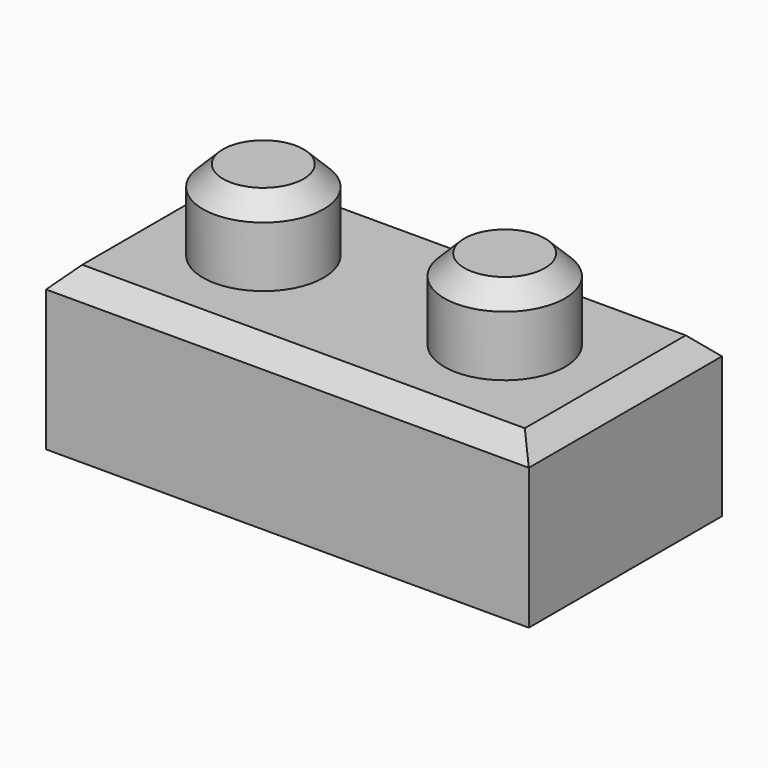
from build123d import *

# Parameters (mm, degrees)
F0_W     = 76.2
F0_H     = 38.1
F1_DEPTH = 25.4
F2_R     = 9.525
F3_DEPTH = 12.7
F4_SIZE2 = 3.175
F4_SIZE  = 3.175
F5_T     = 7.9375


# Not quite as in the source:
# - a shell that OpenCascade refuses in one call is made with other operations: the cavity is built on its own and cut out


with BuildPart() as f1:
    # F0 (on Top) → F1 (new body)
    with BuildSketch(Plane.XY):
        with Locations((38.1, -19.05)):
            Rectangle(F0_W, F0_H)
    extrude(amount=F1_DEPTH)

    # F2 (on face) → F3 (join)
    with BuildSketch(Plane.XY.offset(25.4)):
        with Locations((19.05, -19.05)):
            Circle(F2_R)
        with Locations((57.15, -19.05)):
            Circle(F2_R)
    extrude(amount=F3_DEPTH)

    # F4
    f4_edges = [f1.edges().sort_by_distance(p)[0] for p in [
        (9.525, -19.05, 38.1),
        (47.625, -19.05, 38.1),
        (38.1, -38.1, 25.4),
        (76.2, -19.05, 25.4),
        (0, -19.05, 25.4),
        (38.1, 0, 25.4),
    ]]
    chamfer(f4_edges, length=F4_SIZE, length2=F4_SIZE2)

    # F5: shell of thickness 7.9375, made by hand


with BuildPart() as f5_core1:
    # F5_t2: copy of F1
    add(f1.part)

    # the walls: a layer under each face that stays
    f5_faces = [f5_core1.faces().sort_by_distance(p)[0] for p in [
        (38.1, 0, 11.1125),
        (76.2, -19.05, 11.1125),
        (38.1, -1.5875, 23.8125),
        (0, -19.05, 11.1125),
        (38.1, -38.1, 11.1125),
        (74.6125, -19.05, 23.8125),
        (38.1, -19.05, 25.4),
        (1.5875, -19.05, 23.8125),
        (38.1, -36.5125, 23.8125),
        (9.525, -19.05, 30.1625),
        (47.625, -19.05, 30.1625),
        (11.1125, -19.05, 36.5125),
        (49.2125, -19.05, 36.5125),
        (19.05, -19.05, 38.1),
        (57.15, -19.05, 38.1),
    ]]
    thicken(f5_faces, amount=-F5_T, mode=Mode.SUBTRACT)

    # F5_s3 → F5_t4 (revolve, cut)
    with BuildSketch(Plane.XZ.offset(19.05)):
        Polygon((28.654375, 25.479375), (28.575, 17.4625), (20.6375, 17.4625), (20.6375, 25.4), align=None)
    revolve(axis=Axis((19.05, -19.05, 25.4), (0, 0, 1)), mode=Mode.SUBTRACT)

    # F5_s5 → F5_t6 (revolve, cut)
    with BuildSketch(Plane.XZ.offset(19.05)):
        Polygon((66.754375, 25.479375), (66.675, 17.4625), (58.7375, 17.4625), (58.7375, 25.4), align=None)
    revolve(axis=Axis((57.15, -19.05, 25.4), (0, 0, 1)), mode=Mode.SUBTRACT)


with BuildPart() as f1_1:
    add(f1.part)

    # what is left inside the walls is the cavity
    f5_cavity = [f5_core1.part.solids().sort_by_distance(p)[0] for p in [
        (38.1, -22.754167, 0.079375),
    ]]
    add(f5_cavity, mode=Mode.SUBTRACT)


solid = f1_1.part
